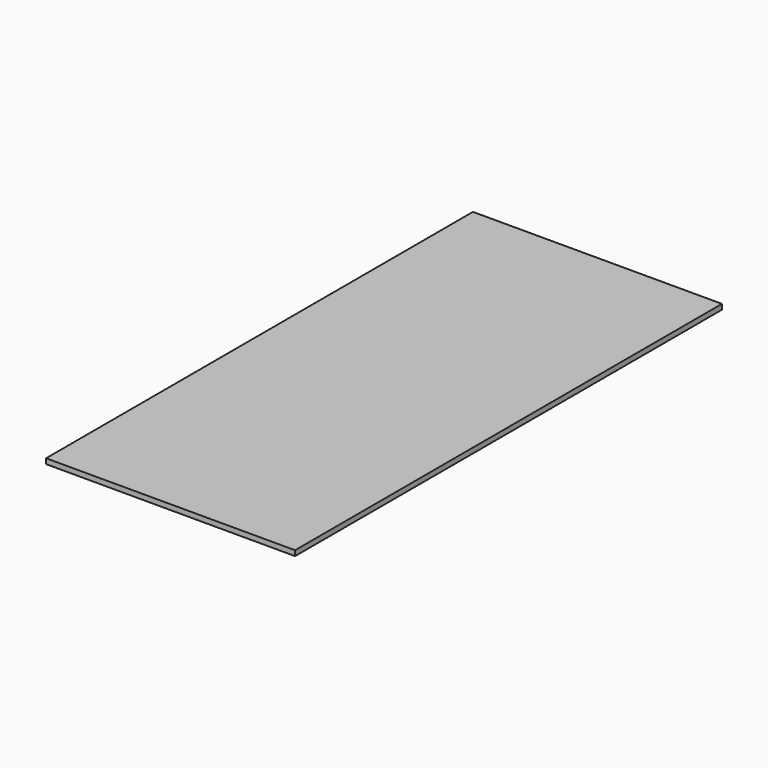
from build123d import *

# Parameters (mm, degrees)
F1_W     = 911.225
F1_H     = 1952.625
F2_DEPTH = 19.05


with BuildPart() as f2:
    # F1 (on Top) → F2 (new body)
    with BuildSketch(Plane.XY):
        with Locations((-0.9625, -0.9625)):
            Rectangle(F1_W, F1_H)
    extrude(amount=F2_DEPTH)


solid = f2.part
